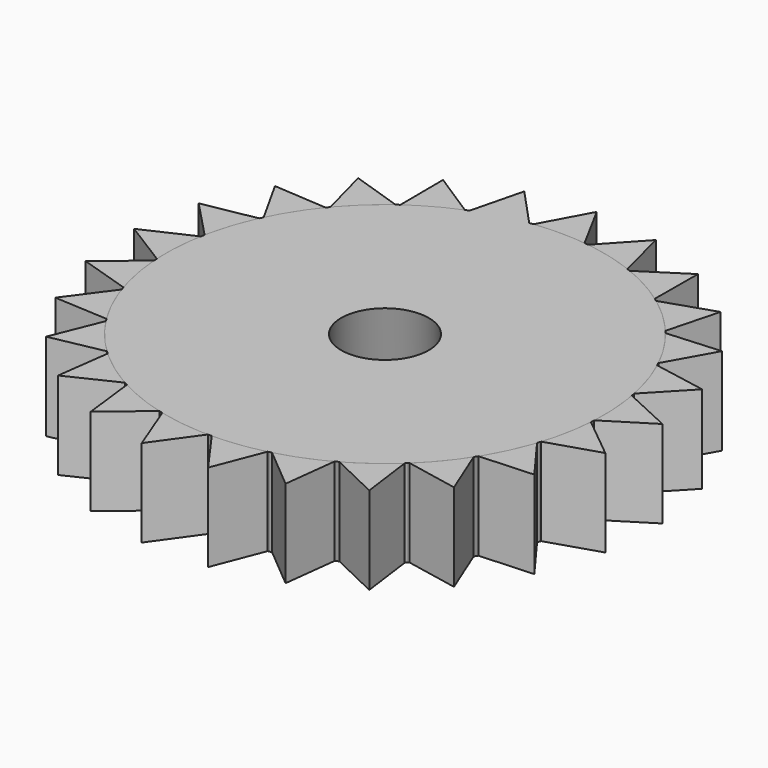
from build123d import *

# Parameters (mm, degrees)
F0_R     = 25
F1_DEPTH = 10
F2_R     = 5
F3_DEPTH = 10.001
F5_DEPTH = 10
F8_COUNT = 25


# Not quite as in the source:
# - a feature names something its author has since deleted; it is built from what else it names


with BuildPart() as f1:
    # F0 (on Top) → F1 (new body)
    with BuildSketch(Plane.XY):
        Circle(F0_R)
    extrude(amount=F1_DEPTH)

    # F2 (on face) → F3 (cut, through all)
    with BuildSketch(Plane.XY.offset(10)):
        Circle(F2_R)
    extrude(amount=-F3_DEPTH, mode=Mode.SUBTRACT)

    # F4 (on Top) → F5 (join)
    with BuildSketch(Plane.XY):
        Polygon((2.9131918618, 24.8296861272), (0, 30.2140377462), (-2.9131918618, 24.8296861272), align=None)
    extrude(amount=F5_DEPTH)


with BuildPart() as f8_1:
    # F8: instance of F1
    add(f1.part.rotate(Axis((0, 0, -0.5598338321), (0, 0, -1)), 1 * 360 / F8_COUNT))


with BuildPart() as f8_2:
    # F8: instance of F1
    add(f1.part.rotate(Axis((0, 0, -0.5598338321), (0, 0, -1)), 2 * 360 / F8_COUNT))


with BuildPart() as f8_3:
    # F8: instance of F1
    add(f1.part.rotate(Axis((0, 0, -0.5598338321), (0, 0, -1)), 3 * 360 / F8_COUNT))


with BuildPart() as f8_4:
    # F8: instance of F1
    add(f1.part.rotate(Axis((0, 0, -0.5598338321), (0, 0, -1)), 4 * 360 / F8_COUNT))


with BuildPart() as f8_5:
    # F8: instance of F1
    add(f1.part.rotate(Axis((0, 0, -0.5598338321), (0, 0, -1)), 5 * 360 / F8_COUNT))


with BuildPart() as f8_6:
    # F8: instance of F1
    add(f1.part.rotate(Axis((0, 0, -0.5598338321), (0, 0, -1)), 6 * 360 / F8_COUNT))


with BuildPart() as f8_7:
    # F8: instance of F1
    add(f1.part.rotate(Axis((0, 0, -0.5598338321), (0, 0, -1)), 7 * 360 / F8_COUNT))


with BuildPart() as f8_8:
    # F8: instance of F1
    add(f1.part.rotate(Axis((0, 0, -0.5598338321), (0, 0, -1)), 8 * 360 / F8_COUNT))


with BuildPart() as f8_9:
    # F8: instance of F1
    add(f1.part.rotate(Axis((0, 0, -0.5598338321), (0, 0, -1)), 9 * 360 / F8_COUNT))


with BuildPart() as f8_10:
    # F8: instance of F1
    add(f1.part.rotate(Axis((0, 0, -0.5598338321), (0, 0, -1)), 10 * 360 / F8_COUNT))


with BuildPart() as f8_11:
    # F8: instance of F1
    add(f1.part.rotate(Axis((0, 0, -0.5598338321), (0, 0, -1)), 11 * 360 / F8_COUNT))


with BuildPart() as f8_12:
    # F8: instance of F1
    add(f1.part.rotate(Axis((0, 0, -0.5598338321), (0, 0, -1)), 12 * 360 / F8_COUNT))


with BuildPart() as f8_13:
    # F8: instance of F1
    add(f1.part.rotate(Axis((0, 0, -0.5598338321), (0, 0, -1)), 13 * 360 / F8_COUNT))


with BuildPart() as f8_14:
    # F8: instance of F1
    add(f1.part.rotate(Axis((0, 0, -0.5598338321), (0, 0, -1)), 14 * 360 / F8_COUNT))


with BuildPart() as f8_15:
    # F8: instance of F1
    add(f1.part.rotate(Axis((0, 0, -0.5598338321), (0, 0, -1)), 15 * 360 / F8_COUNT))


with BuildPart() as f8_16:
    # F8: instance of F1
    add(f1.part.rotate(Axis((0, 0, -0.5598338321), (0, 0, -1)), 16 * 360 / F8_COUNT))


with BuildPart() as f8_17:
    # F8: instance of F1
    add(f1.part.rotate(Axis((0, 0, -0.5598338321), (0, 0, -1)), 17 * 360 / F8_COUNT))


with BuildPart() as f8_18:
    # F8: instance of F1
    add(f1.part.rotate(Axis((0, 0, -0.5598338321), (0, 0, -1)), 18 * 360 / F8_COUNT))


with BuildPart() as f8_19:
    # F8: instance of F1
    add(f1.part.rotate(Axis((0, 0, -0.5598338321), (0, 0, -1)), 19 * 360 / F8_COUNT))


with BuildPart() as f8_20:
    # F8: instance of F1
    add(f1.part.rotate(Axis((0, 0, -0.5598338321), (0, 0, -1)), 20 * 360 / F8_COUNT))


with BuildPart() as f8_21:
    # F8: instance of F1
    add(f1.part.rotate(Axis((0, 0, -0.5598338321), (0, 0, -1)), 21 * 360 / F8_COUNT))


with BuildPart() as f8_22:
    # F8: instance of F1
    add(f1.part.rotate(Axis((0, 0, -0.5598338321), (0, 0, -1)), 22 * 360 / F8_COUNT))


with BuildPart() as f8_23:
    # F8: instance of F1
    add(f1.part.rotate(Axis((0, 0, -0.5598338321), (0, 0, -1)), 23 * 360 / F8_COUNT))


with BuildPart() as f8_24:
    # F8: instance of F1
    add(f1.part.rotate(Axis((0, 0, -0.5598338321), (0, 0, -1)), 24 * 360 / F8_COUNT))


solid = Compound([f1.part, f8_1.part, f8_2.part, f8_3.part, f8_4.part, f8_5.part, f8_6.part, f8_7.part, f8_8.part, f8_9.part, f8_10.part, f8_11.part, f8_12.part, f8_13.part, f8_14.part, f8_15.part, f8_16.part, f8_17.part, f8_18.part, f8_19.part, f8_20.part, f8_21.part, f8_22.part, f8_23.part, f8_24.part])
